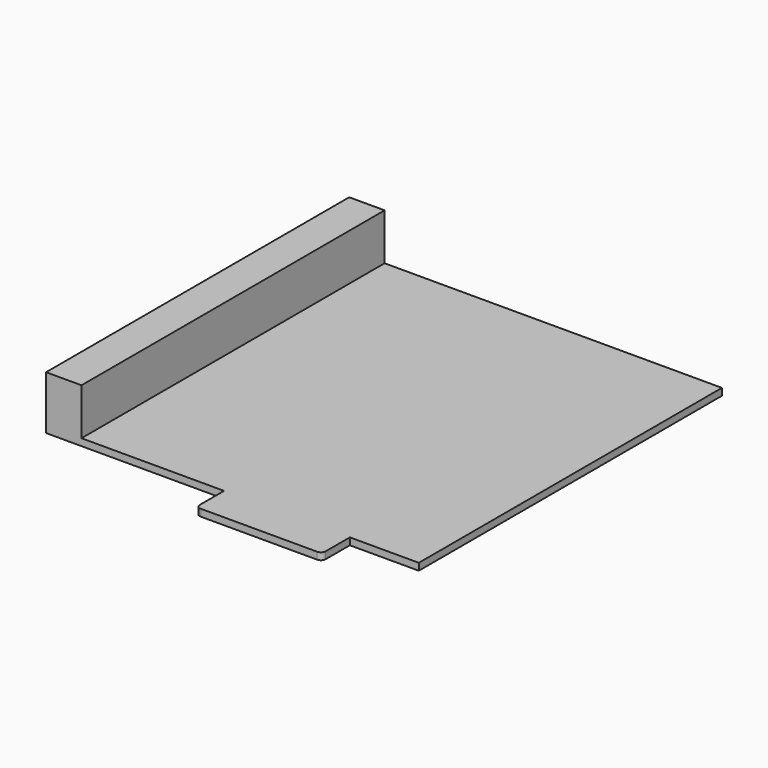
from build123d import *

# Parameters (mm, degrees)
F0_W     = 80
F0_H     = 81.325
F1_DEPTH = 0.75
F3_E1_W  = 27
F3_E1_H  = 1.5
F4_DEPTH = 7.5
F5_R     = 1
F7_W     = 7.6
F7_H     = 81.325
F8_DEPTH = 10


# Not quite as in the source:
# - two fillets or chamfers of one size are made in one step


with BuildPart() as f1:
    # F0 (on Top) → F1 (new body, symmetric)
    with BuildSketch(Plane.XY):
        Rectangle(F0_W, F0_H)
    extrude(amount=F1_DEPTH, both=True)

    # F3_E1 (on explicit) → F4 (join)
    with BuildSketch(Plane(origin=(-1.8, -40.6625, 0.75), x_dir=(1, 0, 0), z_dir=(0, 1, 0))):
        with Locations((13.5, 0.75)):
            Rectangle(F3_E1_W, F3_E1_H)
    extrude(amount=-F4_DEPTH)

    # F5
    f5_edges = [f1.edges().sort_by_distance(p)[0] for p in [
        (-1.8, -48.1625, 0),
        (25.2, -48.1625, 0),
    ]]
    fillet(f5_edges, radius=F5_R)

    # F7 (on face) → F8 (join)
    with BuildSketch(Plane.XY.offset(0.75)):
        with Locations((-36.2, 0)):
            Rectangle(F7_W, F7_H)
    extrude(amount=F8_DEPTH)


solid = f1.part
